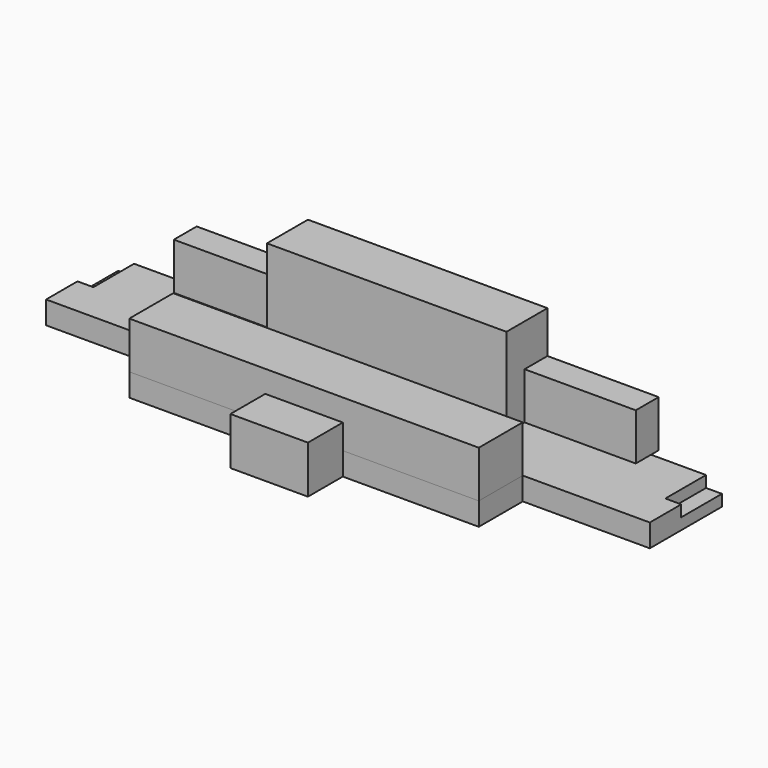
from build123d import *

# Parameters (mm, degrees)
F0_W      = 1418
F0_H      = 358
F1_DEPTH  = 4750
F4_DEPTH  = 1400
F5_DEPTH  = 737
F3_W      = 1220
F3_H      = 686
F6_DEPTH  = 390
F7_DEPTH  = 359
F8_DEPTH  = 359
F10_W     = 250
F10_H     = 179
F11_DEPTH = 800
F3_W_2    = 1750
F3_H_2    = 450
F3_H_3    = 300
F3_H_4    = 150
F12_DEPTH = 737


with BuildPart() as f1:
    # F0 (on Right) → F1 (new body)
    with BuildSketch(Plane.YZ):
        with Locations((-884, -1771)):
            Rectangle(F0_W, F0_H)
    extrude(amount=-F1_DEPTH)


with BuildPart() as f2_1:
    # F2: instance of F1
    add(f1.part.mirror(Plane(origin=(0, -884, -1771), x_dir=(0, 1, 0), z_dir=(1, 0, 0))))


with BuildPart() as f4:
    # F3 (on face) → F4 (new body)
    with BuildSketch(Plane.XY.offset(-1592)):
        Polygon((0, -175), (-1884.5, -175), (-1884.5, -475), (-1884.5, -831), (0, -831), align=None)
        Polygon((1884.5, -475), (1884.5, -25), (-1884.5, -25), (-1884.5, -175), (0, -175), (0, -831), (1884.5, -831), align=None)
    extrude(amount=F4_DEPTH)

    # F3 (on face) → F12 (join)
    with BuildSketch(Plane.XY.offset(-1592)):
        with Locations((2759.5, -250)):
            Rectangle(F3_W_2, F3_H_2)
        with Locations((-2759.5, -325)):
            Rectangle(F3_W_2, F3_H_3)
        with Locations((-2759.5, -100)):
            Rectangle(F3_W_2, F3_H_4)
    extrude(amount=F12_DEPTH)


with BuildPart() as f5:
    # F3 (on face) → F5 (new body)
    with BuildSketch(Plane.XY.offset(-1592)):
        Polygon((2750, -1593), (0, -1593), (-2750, -1593), (-2750, -2457), (-610, -2457), (610, -2457), (2750, -2457), align=None)
    extrude(amount=F5_DEPTH)


with BuildPart() as f6:
    # F3 (on face) → F6 (new body)
    with BuildSketch(Plane.XY.offset(-1592)):
        with Locations((0, -2800)):
            Rectangle(F3_W, F3_H)
    extrude(amount=F6_DEPTH)

    # F3 (on face) → F7 (join)
    with BuildSketch(Plane.XY.offset(-1592)):
        with Locations((0, -2800)):
            Rectangle(F3_W, F3_H)
    extrude(amount=-F7_DEPTH)


with BuildPart() as f1_1:
    add(f1.part)

    add(f2_1.part)  # F8 merges F2_1
    # F3 (on face) → F8 (join)
    with BuildSketch(Plane.XY.offset(-1592)):
        Polygon((2750, -1593), (0, -1593), (-2750, -1593), (-2750, -2457), (-610, -2457), (610, -2457), (2750, -2457), align=None)
    extrude(amount=-F8_DEPTH)

    # F9: union 

    # F10 (on face) → F11 (cut)
    with BuildSketch(Plane(origin=(0, -175, 0), x_dir=(-1, 0, 0), z_dir=(0, 1, 0))):
        with Locations((4625, -1681.5)):
            Rectangle(F10_W, F10_H)
        with Locations((-4625, -1681.5)):
            Rectangle(F10_W, F10_H)
    extrude(amount=-F11_DEPTH, mode=Mode.SUBTRACT)


solid = Compound([f4.part, f5.part, f6.part, f1_1.part])
